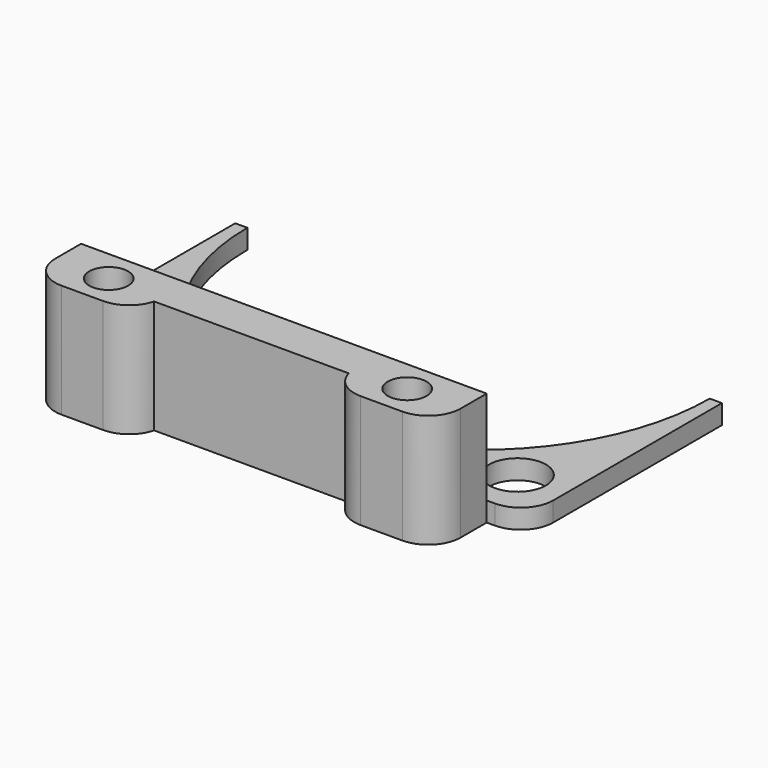
from build123d import *

# Parameters (mm, degrees)
F0_R        = 1.2
F0_W        = 12
F0_H        = 2.5
F0_R_2      = 1.75
F1_DEPTH    = 1.2
F2_DEPTH    = 7
F3_T1_DEPTH = 17
F3_T3_DEPTH = 16.6824583655
F3_T5_DEPTH = 11.2


# Not quite as in the source:
# - a fillet or chamfer that OpenCascade refuses, or shapes differently, is made with other operations: its cross-section is extruded or revolved along the edge and cut away or added
# - a feature names something its author has since deleted; it is built from what else it names


with BuildPart() as f1:
    # F0 (on Top) → F1 (new body)
    with BuildSketch(Plane.XY):
        Polygon((-6, -17.5), (-6, -15), (-12.5, -15), (-12.5, -19), (-6, -19), align=None)
        with Locations((-9.2, -17)):
            Circle(F0_R, mode=Mode.SUBTRACT)
        with Locations((0, -16.25)):
            Rectangle(F0_W, F0_H)
        Polygon((12.5, -19), (12.5, -15), (6, -15), (6, -17.5), (6, -19), align=None)
        with Locations((9.2, -17)):
            Circle(F0_R, mode=Mode.SUBTRACT)
        with BuildLine():
            Line((12.5, -15), (15, -15))
            Line((15, -15), (15, 0))
            Line((15, 0), (14.25, 0))
            ThreePointArc((14.25, 0), (0, -14.25), (-14.25, 0))
            Line((-14.25, 0), (-15, 0))
            Line((-15, 0), (-15, -15))
            Line((-15, -15), (-12.5, -15))
            Line((-12.5, -15), (-6, -15))
            Line((-6, -15), (6, -15))
            Line((6, -15), (12.5, -15))
        make_face()
        with Locations((-12, -12)):
            Circle(F0_R_2, mode=Mode.SUBTRACT)
        with Locations((12, -12)):
            Circle(F0_R_2, mode=Mode.SUBTRACT)
    extrude(amount=F1_DEPTH)

    # F0 (on Top) → F2 (join)
    with BuildSketch(Plane.XY):
        with Locations((0, -16.25)):
            Rectangle(F0_W, F0_H)
        Polygon((-6, -17.5), (-6, -15), (-12.5, -15), (-12.5, -19), (-6, -19), align=None)
        with Locations((-9.2, -17)):
            Circle(F0_R, mode=Mode.SUBTRACT)
        Polygon((12.5, -19), (12.5, -15), (6, -15), (6, -17.5), (6, -19), align=None)
        with Locations((9.2, -17)):
            Circle(F0_R, mode=Mode.SUBTRACT)
    extrude(amount=F2_DEPTH)

    # F3: fillet of radius 2 on 6 edges, made by hand

    # F3_s2 → F3_t1 (cut)
    with BuildSketch(Plane.XY.offset(-5)):
        with BuildLine():
            ThreePointArc((-12.5, -17), (-11.9142135624, -18.4142135624), (-10.5, -19))
            Line((-10.5, -19), (-12.5, -19))
            Line((-12.5, -19), (-12.5, -17))
        make_face()
        with BuildLine():
            ThreePointArc((10.5, -19), (11.9142135624, -18.4142135624), (12.5, -17))
            Line((12.5, -17), (12.5, -19))
            Line((12.5, -19), (10.5, -19))
        make_face()
    extrude(amount=F3_T1_DEPTH, mode=Mode.SUBTRACT)

    # F3_s4 → F3_t3 (cut)
    with BuildSketch(Plane.XY.offset(-4.8412291828)):
        with BuildLine():
            ThreePointArc((-6, -17.5), (-6.7117468017, -18.5811388301), (-7.9364916731, -19))
            Line((-7.9364916731, -19), (-6, -19))
            Line((-6, -19), (-6, -17.5))
        make_face()
        with BuildLine():
            ThreePointArc((7.9364916731, -19), (6.7117468017, -18.5811388301), (6, -17.5))
            Line((6, -17.5), (6, -19))
            Line((6, -19), (7.9364916731, -19))
        make_face()
    extrude(amount=F3_T3_DEPTH, mode=Mode.SUBTRACT)

    # F3_s6 → F3_t5 (cut)
    with BuildSketch(Plane.XY.offset(-5)):
        with BuildLine():
            ThreePointArc((15, -13), (14.4142135624, -14.4142135624), (13, -15))
            Line((13, -15), (15, -15))
            Line((15, -15), (15, -13))
        make_face()
        with BuildLine():
            ThreePointArc((-15, -13), (-14.4142135624, -14.4142135624), (-13, -15))
            Line((-13, -15), (-15, -15))
            Line((-15, -15), (-15, -13))
        make_face()
    extrude(amount=F3_T5_DEPTH, mode=Mode.SUBTRACT)


solid = f1.part
